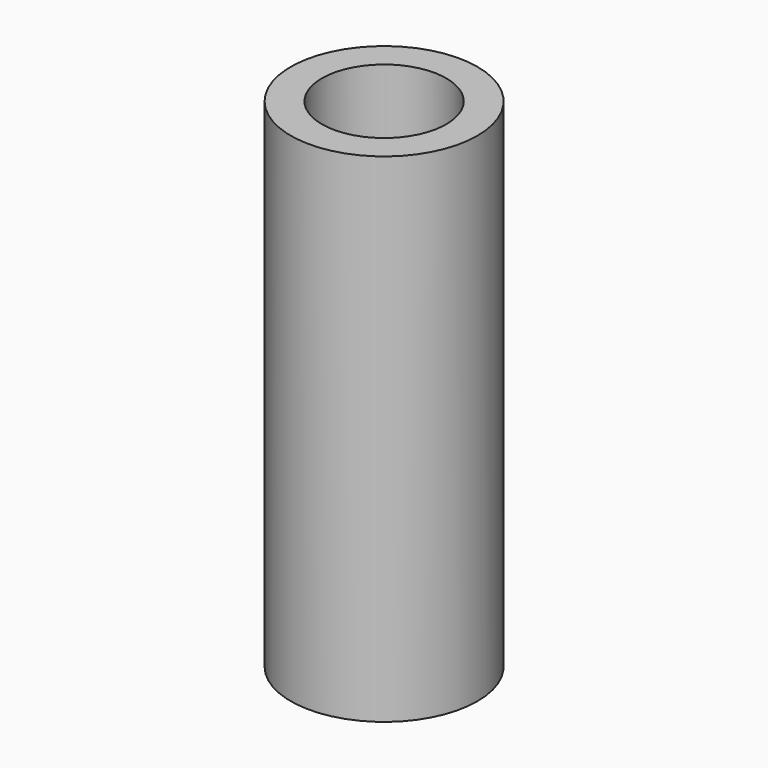
from build123d import *

# Parameters (mm, degrees)
F0_R     = 15
F1_DEPTH = 80
F3_D     = 20


# Not quite as in the source:
# - the program builds the solid bodies; features that only make, move or delete a surface that nothing else refers to are left out


with BuildPart() as f1:
    # F0 (on Top) → F1 (new body)
    with BuildSketch(Plane.XY):
        Circle(F0_R)
    extrude(amount=F1_DEPTH)

    # F3 (through all)
    with Locations(Plane(origin=(0, 0, 0), x_dir=(1, 0, 0), z_dir=(0, 0, -1))):
        with Locations((0, 0)):
            Hole(F3_D / 2)


solid = f1.part
